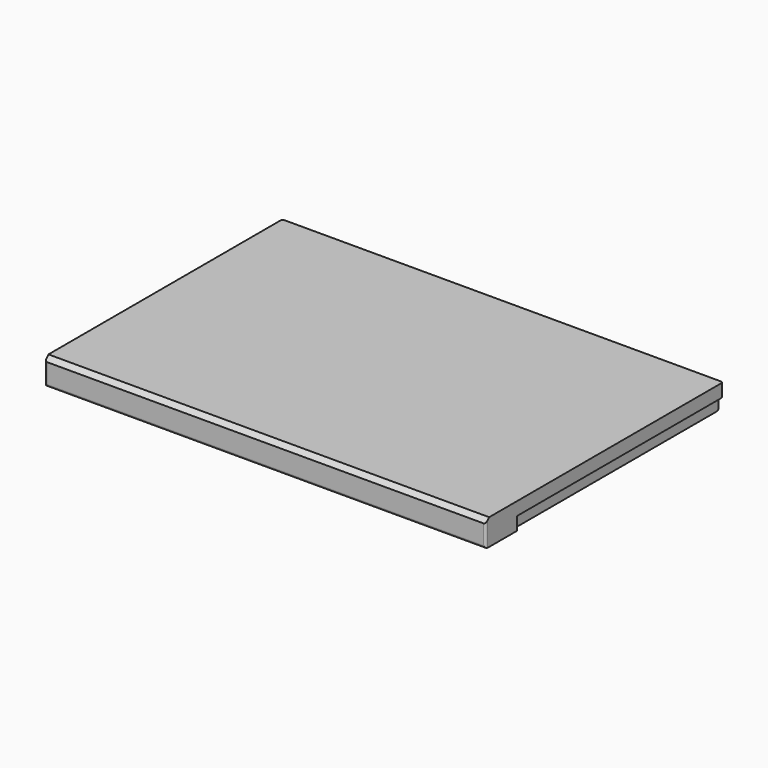
from build123d import *

# Parameters (mm, degrees)
F0_W     = 641.35
F0_H     = 431.8
F1_DEPTH = 38.1
F2_W     = 6.35
F2_H     = 19.05
F3_DEPTH = 431.801
F4_DEPTH = 57.15
F5_SIZE  = 6.35
F7_DEPTH = 12.7
F8_R     = 3.175


with BuildPart() as f1:
    # F0 (on Top) → F1 (new body)
    with BuildSketch(Plane.XY):
        with Locations((320.675, 215.9)):
            Rectangle(F0_W, F0_H)
    extrude(amount=F1_DEPTH)

    # F2 (on face) → F3 (cut, through all)
    with BuildSketch(Plane.XZ):
        with Locations((3.175, 9.525)):
            Rectangle(F2_W, F2_H)
        with Locations((638.175, 9.525)):
            Rectangle(F2_W, F2_H)
    extrude(amount=-F3_DEPTH, mode=Mode.SUBTRACT)

    # F2 (on face) → F4 (join)
    with BuildSketch(Plane.XZ):
        with Locations((3.175, 9.525)):
            Rectangle(F2_W, F2_H)
        with Locations((638.175, 9.525)):
            Rectangle(F2_W, F2_H)
    extrude(amount=-F4_DEPTH)

    # F5
    f5_edges = [f1.edges().sort_by_distance(p)[0] for p in [
        (320.675, 0, 38.1),
    ]]
    chamfer(f5_edges, length=F5_SIZE)

    # F6 (on face) → F7 (cut)
    with BuildSketch(Plane(origin=(0, 0, 0), x_dir=(1, 0, 0), z_dir=(0, 0, -1))):
        with BuildLine():
            Line((577.85, -19.05), (63.5, -19.05))
            ThreePointArc((63.5, -19.05), (57.15, -25.4), (63.5, -31.75))
            Line((63.5, -31.75), (577.85, -31.75))
            ThreePointArc((577.85, -31.75), (584.2, -25.4), (577.85, -19.05))
        make_face()
    extrude(amount=-F7_DEPTH, mode=Mode.SUBTRACT)

    # F8
    f8_edges = [f1.edges().sort_by_distance(p)[0] for p in [
        (0, 0, 15.875),
        (320.675, 0, 0),
        (641.35, 0, 15.875),
        (320.675, 431.8, 0),
        (57.15, 25.4, 0),
        (57.15, 25.4, 12.7),
        (0, 431.8, 28.575),
        (641.35, 431.8, 28.575),
        (320.675, 19.05, 0),
        (320.675, 31.75, 0),
        (584.2, 25.4, 0),
        (320.675, 19.05, 12.7),
        (320.675, 31.75, 12.7),
        (584.2, 25.4, 12.7),
    ]]
    fillet(f8_edges, radius=F8_R)


solid = f1.part
